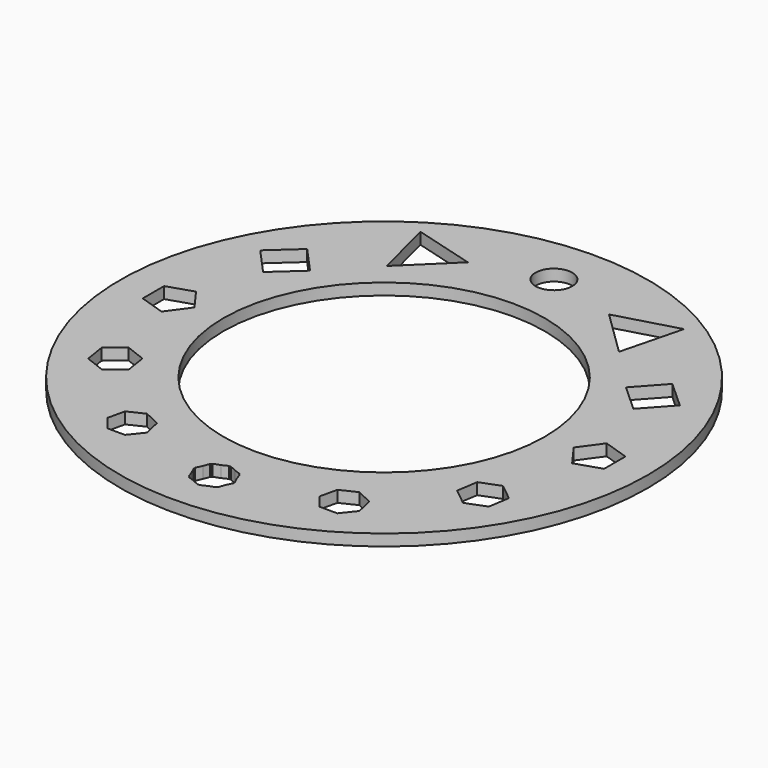
from build123d import *

# Parameters (mm, degrees)
F0_R     = 115
F0_R_2   = 70
F1_DEPTH = 5
F2_R     = 8
F3_DEPTH = 25


with BuildPart() as f1:
    # F0 (on Top) → F1 (new body)
    with BuildSketch(Plane.XY):
        Circle(F0_R)
        Circle(F0_R_2, mode=Mode.SUBTRACT)
    extrude(amount=F1_DEPTH)

    # F2 (on face) → F3 (cut)
    with BuildSketch(Plane.XY.offset(5)):
        with Locations((0, 92.5)):
            Circle(F2_R)
        Polygon((30.7451541874, 84.0570025344), (42.1222582105, 72.9578913502), (50.5819233456, 64.7049331524), (57.422922467, 91.5601138634), align=None)
        Polygon((68.8072985361, 45.6942659799), (72.8301810847, 42.0485246544), (80.6630838702, 34.949948686), (91.4074011641, 46.8057340201), (79.55161583, 57.550051314), align=None)
        Polygon((100.5, -5.812340224), (100.5, 5.812340224), (89.44427191, 9.4045640367), (82.61145618, 0), (89.44427191, -9.4045640367), align=None)
        Polygon((78.6682453406, -55.374818439), (87.2901221684, -52.0587102834), (88.7292266779, -42.9338918444), (81.5464543596, -37.125181561), (72.9245775317, -40.4412897166), (71.4854730222, -49.5661081556), align=None)
        Polygon((42.3974030495, -88.1073498501), (50.1025969505, -88.1073498501), (54.906706769, -82.0831866798), (53.1921398259, -74.571178077), (46.25, -71.2280197367), (39.3078601741, -74.571178077), (37.593293231, -82.0831866798), align=None)
        Polygon((3.065005288, -99.899577335), (5.8217626423, -98.9099722116), (6.010291359, -98.510291359), align=None)
        Polygon((0.4159269752, -101.1491426608), (3.065005288, -99.899577335), (0, -100.9998355537), align=None)
        Polygon((0, -100.9998355537), (3.065005288, -99.899577335), (6.010291359, -98.510291359), (7.399577335, -95.565005288), (8.4998355537, -92.5), (7.399577335, -89.434994712), (6.010291359, -86.489708641), (3.065005288, -85.100422665), (0, -84.0001644463), (-3.065005288, -85.100422665), (-6.010291359, -86.489708641), (-7.399577335, -89.434994712), (-8.4998355537, -92.5), (-7.399577335, -95.565005288), (-6.010291359, -98.510291359), (-3.065005288, -99.899577335), align=None)
        Polygon((7.399577335, -95.565005288), (6.010291359, -98.510291359), (6.4099722116, -98.3217626423), align=None)
        Polygon((-0.4159269752, -101.1491426608), (0, -100.9998355537), (-3.065005288, -99.899577335), align=None)
        Polygon((8.4998355537, -92.5), (7.399577335, -95.565005288), (8.6491426608, -92.9159269752), align=None)
        Polygon((-5.8217626423, -98.9099722116), (-3.065005288, -99.899577335), (-6.010291359, -98.510291359), align=None)
        Polygon((7.399577335, -89.434994712), (8.4998355537, -92.5), (8.6491426608, -92.0840730248), align=None)
        Polygon((-6.4099722116, -98.3217626423), (-6.010291359, -98.510291359), (-7.399577335, -95.565005288), align=None)
        Polygon((6.010291359, -86.489708641), (7.399577335, -89.434994712), (6.4099722116, -86.6782373577), align=None)
        Polygon((-8.6491426608, -92.9159269752), (-7.399577335, -95.565005288), (-8.4998355537, -92.5), align=None)
        Polygon((3.065005288, -85.100422665), (6.010291359, -86.489708641), (5.8217626423, -86.0900277884), align=None)
        Polygon((-8.6491426608, -92.0840730248), (-8.4998355537, -92.5), (-7.399577335, -89.434994712), align=None)
        Polygon((0, -84.0001644463), (3.065005288, -85.100422665), (0.4159269752, -83.8508573392), align=None)
        Polygon((-6.4099722116, -86.6782373577), (-7.399577335, -89.434994712), (-6.010291359, -86.489708641), align=None)
        Polygon((-3.065005288, -85.100422665), (0, -84.0001644463), (-0.4159269752, -83.8508573392), align=None)
        Polygon((-5.8217626423, -86.0900277884), (-6.010291359, -86.489708641), (-3.065005288, -85.100422665), align=None)
        Polygon((-57.422922467, 91.5601138634), (-50.5819233456, 64.7049331524), (-30.7451541874, 84.0570025344), align=None)
        Polygon((-80.6630838702, 34.949948686), (-68.8072985361, 45.6942659799), (-79.55161583, 57.550051314), (-91.4074011641, 46.8057340201), align=None)
        Polygon((-100.5, -5.812340224), (-89.44427191, -9.4045640367), (-82.61145618, 0), (-89.44427191, 9.4045640367), (-100.5, 5.812340224), align=None)
        Polygon((-71.4854730222, -49.5661081556), (-72.9245775317, -40.4412897166), (-81.5464543596, -37.125181561), (-88.7292266779, -42.9338918444), (-87.2901221684, -52.0587102834), (-78.6682453406, -55.374818439), align=None)
        Polygon((-50.1025969505, -88.1073498501), (-42.3974030495, -88.1073498501), (-37.593293231, -82.0831866798), (-39.3078601741, -74.571178077), (-46.25, -71.2280197367), (-53.1921398259, -74.571178077), (-54.906706769, -82.0831866798), align=None)
    extrude(amount=-F3_DEPTH, mode=Mode.SUBTRACT)


solid = f1.part
